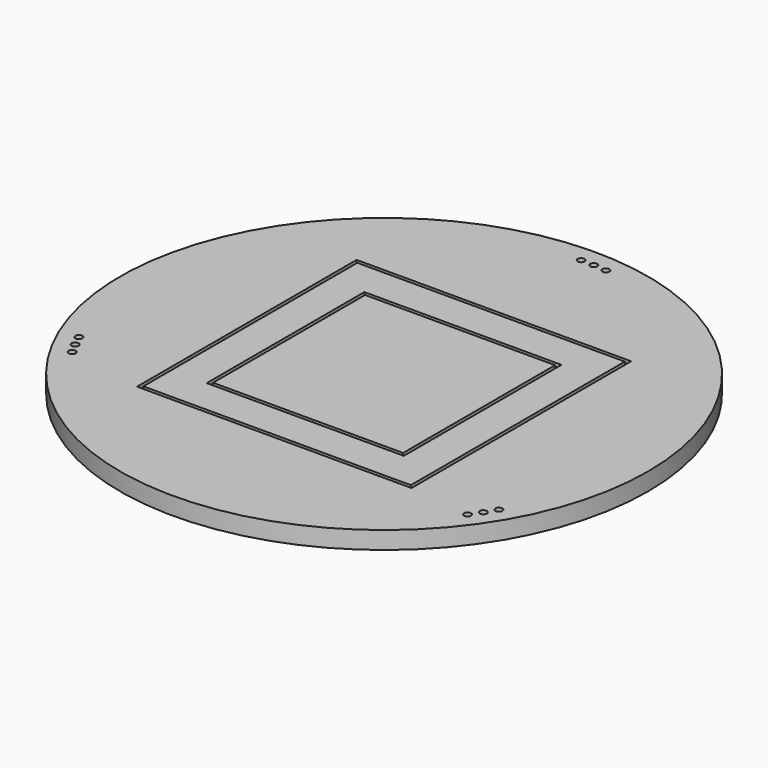
from build123d import *

# Parameters (mm, degrees)
F0_R            = 75
F1_DEPTH        = 5
F2_W            = 78
F2_H            = 78
F2_W_2          = 76
F2_H_2          = 76
F2_W_3          = 56
F2_H_3          = 56
F2_W_4          = 54
F2_H_4          = 54
F3_DEPTH        = 1
F4_R            = 1
F5_DEPTH        = 5.001
F5_COPIES_COUNT = 3


# Not quite as in the source:
# - a pattern or mirror of a feature is missing from the dataset's text; its kind, count and spacing are read off the source's solid


with BuildPart() as f1:
    # F0 (on Top) → F1 (new body)
    with BuildSketch(Plane.XY):
        Circle(F0_R)
    extrude(amount=F1_DEPTH)

    # F2 (on face) → F3 (cut)
    with BuildSketch(Plane.XY.offset(5)):
        Rectangle(F2_W, F2_H)
        Rectangle(F2_W_2, F2_H_2, mode=Mode.SUBTRACT)
        Rectangle(F2_W_3, F2_H_3)
        Rectangle(F2_W_4, F2_H_4, mode=Mode.SUBTRACT)
    extrude(amount=-F3_DEPTH, mode=Mode.SUBTRACT)

    # F4 (on face) → F5 (cut, through all)
    with BuildSketch(Plane.XY.offset(5)):
        with Locations((0, 70)):
            Circle(F4_R)
        with Locations((3.663516937, 69.9040674328)):
            Circle(F4_R)
        with Locations((7.3169924287, 69.6165326758)):
            Circle(F4_R)
    f5 = extrude(amount=-F5_DEPTH, mode=Mode.SUBTRACT)

    # F5_copies: F5 ×3 about axis
    f5_copies_axis = Axis((0, 0, 0), (0, 0, 1))
    for i in range(1, F5_COPIES_COUNT):
        add(f5.rotate(f5_copies_axis, i * 360 / F5_COPIES_COUNT), mode=Mode.SUBTRACT)


solid = f1.part
